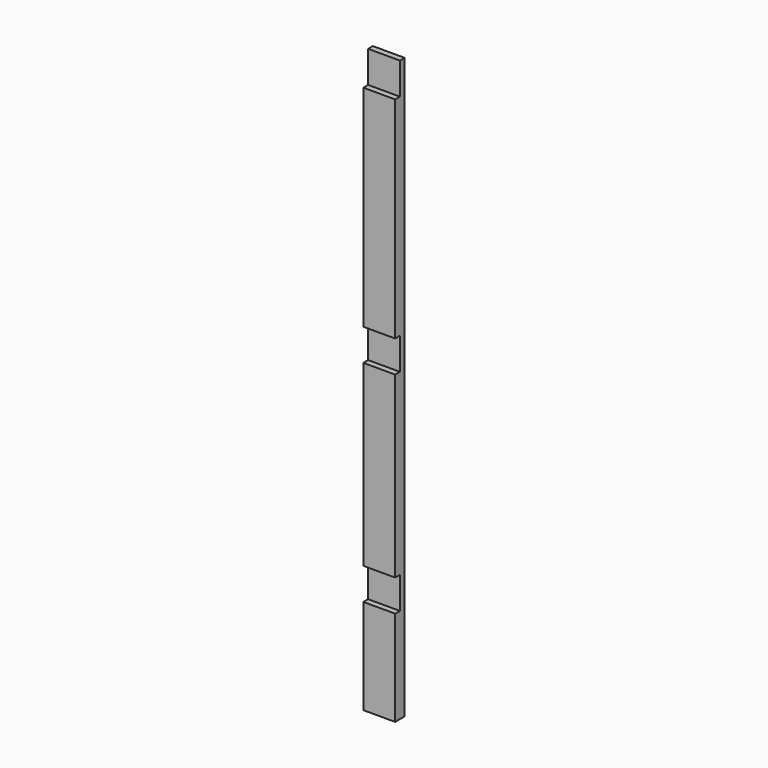
from build123d import *

# Parameters (mm, degrees)
F0_W     = 50.8
F0_H     = 19.05
F1_DEPTH = 927.1
F2_W     = 122.43557321
F2_H     = 50.8
F2_W_2   = 343.1604206562
F2_W_3   = 181.214183569
F3_DEPTH = 25.4


# Not quite as in the source:
# - a feature names something its author has since deleted; it is built from what else it names


with BuildPart() as f1:
    # F0 (on Top) → F1 (new body)
    with BuildSketch(Plane.XY):
        Rectangle(F0_W, F0_H)
    extrude(amount=F1_DEPTH)

    # F2 (on Front) → F3 (cut)
    with BuildSketch(Plane.XZ):
        with Locations((22.4465244144, 177.8)):
            Rectangle(F2_W, F2_H)
        with Locations((-38.7818217278, 901.7)):
            Rectangle(F2_W_2, F2_H)
        with Locations((-23.9842385054, 514.35)):
            Rectangle(F2_W_3, F2_H)
    extrude(amount=F3_DEPTH, mode=Mode.SUBTRACT)


solid = f1.part
